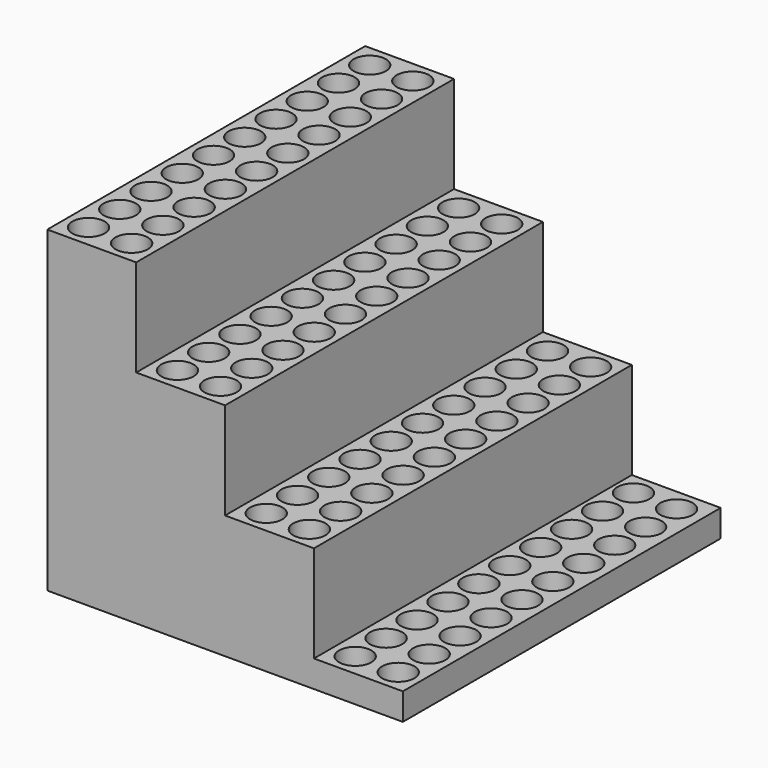
from build123d import *

# Parameters (mm, degrees)
F1_DEPTH  = 295
F2_R      = 12
F3_DEPTH  = 18
F4_R      = 12
F5_DEPTH  = 18
F6_R      = 12
F7_DEPTH  = 18
F8_R      = 12
F9_DEPTH  = 18
F11_DEPTH = 180
F13_DEPTH = 116
F15_DEPTH = 50
F16_DEPTH = 50
F17_DEPTH = 116
F18_DEPTH = 182


# Not quite as in the source:
# - a feature names something its author has since deleted; it is built from what else it names


with BuildPart() as f1:
    # F0 (on Front) → F1 (new body)
    with BuildSketch(Plane.XZ):
        Polygon((-130.714428395, 109.3473359393), (-130.714428395, -126.6526640607), (133.285571605, -126.6526640607), (133.285571605, -106.6526640607), (67.285571605, -106.6526640607), (67.285571605, -34.6526640607), (1.285571605, -34.6526640607), (1.285571605, 37.3473359393), (-64.714428395, 37.3473359393), (-64.714428395, 109.3473359393), align=None)
    extrude(amount=F1_DEPTH)

    # F2 (on face) → F3 (cut)
    with BuildSketch(Plane.XY.offset(-106.6526640607)):
        with Locations((84.285571605, -278)):
            Circle(F2_R)
        with Locations((84.0420044155, -249.0010228624)):
            Circle(F2_R)
        with Locations((83.7984372259, -220.0020457249)):
            Circle(F2_R)
        with Locations((83.5548700364, -191.0030685873)):
            Circle(F2_R)
        with Locations((83.3113028469, -162.0040914498)):
            Circle(F2_R)
        with Locations((83.0677356574, -133.0051143122)):
            Circle(F2_R)
        with Locations((82.8241684679, -104.0061371747)):
            Circle(F2_R)
        with Locations((82.5806012783, -75.0071600371)):
            Circle(F2_R)
        with Locations((82.3370340888, -46.0081828996)):
            Circle(F2_R)
        with Locations((82.0934668993, -17.009205762)):
            Circle(F2_R)
        with Locations((114.0934668993, -17.009205762)):
            Circle(F2_R)
        with Locations((114.3370340888, -46.0081828996)):
            Circle(F2_R)
        with Locations((114.5806012783, -75.0071600371)):
            Circle(F2_R)
        with Locations((114.8241684679, -104.0061371747)):
            Circle(F2_R)
        with Locations((115.0677356574, -133.0051143122)):
            Circle(F2_R)
        with Locations((115.3113028469, -162.0040914498)):
            Circle(F2_R)
        with Locations((115.5548700364, -191.0030685873)):
            Circle(F2_R)
        with Locations((115.7984372259, -220.0020457249)):
            Circle(F2_R)
        with Locations((116.0420044155, -249.0010228624)):
            Circle(F2_R)
        with Locations((116.285571605, -278)):
            Circle(F2_R)
    extrude(amount=-F3_DEPTH, mode=Mode.SUBTRACT)

    # F4 (on face) → F5 (cut)
    with BuildSketch(Plane.XY.offset(-34.6526640607)):
        with Locations((18.285571605, -278)):
            Circle(F4_R)
        with Locations((18.285571605, -249)):
            Circle(F4_R)
        with Locations((18.285571605, -220)):
            Circle(F4_R)
        with Locations((18.285571605, -191)):
            Circle(F4_R)
        with Locations((18.285571605, -162)):
            Circle(F4_R)
        with Locations((18.285571605, -133)):
            Circle(F4_R)
        with Locations((18.285571605, -104)):
            Circle(F4_R)
        with Locations((18.285571605, -75)):
            Circle(F4_R)
        with Locations((18.285571605, -46)):
            Circle(F4_R)
        with Locations((18.285571605, -17)):
            Circle(F4_R)
        with Locations((50.285571605, -17)):
            Circle(F4_R)
        with Locations((50.285571605, -46)):
            Circle(F4_R)
        with Locations((50.285571605, -75)):
            Circle(F4_R)
        with Locations((50.285571605, -104)):
            Circle(F4_R)
        with Locations((50.285571605, -133)):
            Circle(F4_R)
        with Locations((50.285571605, -162)):
            Circle(F4_R)
        with Locations((50.285571605, -191)):
            Circle(F4_R)
        with Locations((50.285571605, -220)):
            Circle(F4_R)
        with Locations((50.285571605, -249)):
            Circle(F4_R)
        with Locations((50.285571605, -278)):
            Circle(F4_R)
    extrude(amount=-F5_DEPTH, mode=Mode.SUBTRACT)

    # F6 (on face) → F7 (cut)
    with BuildSketch(Plane.XY.offset(37.3473359393)):
        with Locations((-47.714428395, -278)):
            Circle(F6_R)
        with Locations((-47.714428395, -249)):
            Circle(F6_R)
        with Locations((-47.714428395, -220)):
            Circle(F6_R)
        with Locations((-47.714428395, -191)):
            Circle(F6_R)
        with Locations((-47.714428395, -162)):
            Circle(F6_R)
        with Locations((-47.714428395, -133)):
            Circle(F6_R)
        with Locations((-47.714428395, -104)):
            Circle(F6_R)
        with Locations((-47.714428395, -75)):
            Circle(F6_R)
        with Locations((-47.714428395, -46)):
            Circle(F6_R)
        with Locations((-47.714428395, -17)):
            Circle(F6_R)
        with Locations((-15.714428395, -17)):
            Circle(F6_R)
        with Locations((-15.714428395, -46)):
            Circle(F6_R)
        with Locations((-15.714428395, -75)):
            Circle(F6_R)
        with Locations((-15.714428395, -104)):
            Circle(F6_R)
        with Locations((-15.714428395, -133)):
            Circle(F6_R)
        with Locations((-15.714428395, -162)):
            Circle(F6_R)
        with Locations((-15.714428395, -191)):
            Circle(F6_R)
        with Locations((-15.714428395, -220)):
            Circle(F6_R)
        with Locations((-15.714428395, -249)):
            Circle(F6_R)
        with Locations((-15.714428395, -278)):
            Circle(F6_R)
    extrude(amount=-F7_DEPTH, mode=Mode.SUBTRACT)

    # F8 (on face) → F9 (cut)
    with BuildSketch(Plane.XY.offset(109.3473359393)):
        with Locations((-113.714428395, -278)):
            Circle(F8_R)
        with Locations((-113.714428395, -249)):
            Circle(F8_R)
        with Locations((-113.714428395, -220)):
            Circle(F8_R)
        with Locations((-113.714428395, -191)):
            Circle(F8_R)
        with Locations((-113.714428395, -162)):
            Circle(F8_R)
        with Locations((-113.714428395, -133)):
            Circle(F8_R)
        with Locations((-113.714428395, -104)):
            Circle(F8_R)
        with Locations((-113.714428395, -75)):
            Circle(F8_R)
        with Locations((-113.714428395, -46)):
            Circle(F8_R)
        with Locations((-113.714428395, -17)):
            Circle(F8_R)
        with Locations((-81.714428395, -17)):
            Circle(F8_R)
        with Locations((-81.714428395, -46)):
            Circle(F8_R)
        with Locations((-81.714428395, -75)):
            Circle(F8_R)
        with Locations((-81.714428395, -104)):
            Circle(F8_R)
        with Locations((-81.714428395, -133)):
            Circle(F8_R)
        with Locations((-81.714428395, -162)):
            Circle(F8_R)
        with Locations((-81.714428395, -191)):
            Circle(F8_R)
        with Locations((-81.714428395, -220)):
            Circle(F8_R)
        with Locations((-81.714428395, -249)):
            Circle(F8_R)
        with Locations((-81.714428395, -278)):
            Circle(F8_R)
    extrude(amount=-F9_DEPTH, mode=Mode.SUBTRACT)

    # F10 (on face) → F11 (cut)
    with BuildSketch(Plane(origin=(-130.714428395, 0, 0), x_dir=(0, -1, 0), z_dir=(-1, 0, 0))):
        with BuildLine():
            ThreePointArc((7.2532056552, -79.6526640607), (17, -84.6526640607), (26.7467943448, -79.6526640607))
            ThreePointArc((26.7467943448, -79.6526640607), (17, -74.6526640607), (7.2532056552, -79.6526640607))
        make_face()
        with BuildLine():
            ThreePointArc((7.2532056552, -79.6526640607), (13.3231489109, -98.0754818422), (29, -86.6526640607))
            ThreePointArc((29, -86.6526640607), (28.4228177815, -82.9758129716), (26.7467943448, -79.6526640607))
            ThreePointArc((26.7467943448, -79.6526640607), (17, -84.6526640607), (7.2532056552, -79.6526640607))
        make_face()
        with BuildLine():
            ThreePointArc((36.2532056552, -79.6526640607), (46, -84.6526640607), (55.7467943448, -79.6526640607))
            ThreePointArc((55.7467943448, -79.6526640607), (46, -74.6526640607), (36.2532056552, -79.6526640607))
        make_face()
        with BuildLine():
            ThreePointArc((36.2532056552, -79.6526640607), (42.3231489109, -98.0754818422), (58, -86.6526640607))
            ThreePointArc((58, -86.6526640607), (57.4228177815, -82.9758129716), (55.7467943448, -79.6526640607))
            ThreePointArc((55.7467943448, -79.6526640607), (46, -84.6526640607), (36.2532056552, -79.6526640607))
        make_face()
        with BuildLine():
            ThreePointArc((65.2532056552, -79.6526640607), (75, -84.6526640607), (84.7467943448, -79.6526640607))
            ThreePointArc((84.7467943448, -79.6526640607), (75, -74.6526640607), (65.2532056552, -79.6526640607))
        make_face()
        with BuildLine():
            ThreePointArc((65.2532056552, -79.6526640607), (71.3231489109, -98.0754818422), (87, -86.6526640607))
            ThreePointArc((87, -86.6526640607), (86.4228177815, -82.9758129716), (84.7467943448, -79.6526640607))
            ThreePointArc((84.7467943448, -79.6526640607), (75, -84.6526640607), (65.2532056552, -79.6526640607))
        make_face()
        with BuildLine():
            ThreePointArc((94.2532056552, -79.6526640607), (104, -84.6526640607), (113.7467943448, -79.6526640607))
            ThreePointArc((113.7467943448, -79.6526640607), (104, -74.6526640607), (94.2532056552, -79.6526640607))
        make_face()
        with BuildLine():
            ThreePointArc((94.2532056552, -79.6526640607), (100.3231489109, -98.0754818422), (116, -86.6526640607))
            ThreePointArc((116, -86.6526640607), (115.4228177815, -82.9758129716), (113.7467943448, -79.6526640607))
            ThreePointArc((113.7467943448, -79.6526640607), (104, -84.6526640607), (94.2532056552, -79.6526640607))
        make_face()
        with BuildLine():
            ThreePointArc((123.2532056552, -79.6526640607), (133, -84.6526640607), (142.7467943448, -79.6526640607))
            ThreePointArc((142.7467943448, -79.6526640607), (133, -74.6526640607), (123.2532056552, -79.6526640607))
        make_face()
        with BuildLine():
            ThreePointArc((123.2532056552, -79.6526640607), (129.3231489109, -98.0754818422), (145, -86.6526640607))
            ThreePointArc((145, -86.6526640607), (144.4228177815, -82.9758129716), (142.7467943448, -79.6526640607))
            ThreePointArc((142.7467943448, -79.6526640607), (133, -84.6526640607), (123.2532056552, -79.6526640607))
        make_face()
        with BuildLine():
            ThreePointArc((152.2532056552, -79.6526640607), (162, -84.6526640607), (171.7467943448, -79.6526640607))
            ThreePointArc((171.7467943448, -79.6526640607), (162, -74.6526640607), (152.2532056552, -79.6526640607))
        make_face()
        with BuildLine():
            ThreePointArc((152.2532056552, -79.6526640607), (158.3231489109, -98.0754818422), (174, -86.6526640607))
            ThreePointArc((174, -86.6526640607), (173.4228177815, -82.9758129716), (171.7467943448, -79.6526640607))
            ThreePointArc((171.7467943448, -79.6526640607), (162, -84.6526640607), (152.2532056552, -79.6526640607))
        make_face()
        with BuildLine():
            ThreePointArc((181.2532056552, -79.6526640607), (191, -84.6526640607), (200.7467943448, -79.6526640607))
            ThreePointArc((200.7467943448, -79.6526640607), (191, -74.6526640607), (181.2532056552, -79.6526640607))
        make_face()
        with BuildLine():
            ThreePointArc((181.2532056552, -79.6526640607), (187.3231489109, -98.0754818422), (203, -86.6526640607))
            ThreePointArc((203, -86.6526640607), (202.4228177815, -82.9758129716), (200.7467943448, -79.6526640607))
            ThreePointArc((200.7467943448, -79.6526640607), (191, -84.6526640607), (181.2532056552, -79.6526640607))
        make_face()
        with BuildLine():
            ThreePointArc((210.2532056552, -79.6526640607), (220, -84.6526640607), (229.7467943448, -79.6526640607))
            ThreePointArc((229.7467943448, -79.6526640607), (220, -74.6526640607), (210.2532056552, -79.6526640607))
        make_face()
        with BuildLine():
            ThreePointArc((210.2532056552, -79.6526640607), (216.3231489109, -98.0754818422), (232, -86.6526640607))
            ThreePointArc((232, -86.6526640607), (231.4228177815, -82.9758129716), (229.7467943448, -79.6526640607))
            ThreePointArc((229.7467943448, -79.6526640607), (220, -84.6526640607), (210.2532056552, -79.6526640607))
        make_face()
        with BuildLine():
            ThreePointArc((239.2532056552, -79.6526640607), (249, -84.6526640607), (258.7467943448, -79.6526640607))
            ThreePointArc((258.7467943448, -79.6526640607), (249, -74.6526640607), (239.2532056552, -79.6526640607))
        make_face()
        with BuildLine():
            ThreePointArc((239.2532056552, -79.6526640607), (245.3231489109, -98.0754818422), (261, -86.6526640607))
            ThreePointArc((261, -86.6526640607), (260.4228177815, -82.9758129716), (258.7467943448, -79.6526640607))
            ThreePointArc((258.7467943448, -79.6526640607), (249, -84.6526640607), (239.2532056552, -79.6526640607))
        make_face()
        with BuildLine():
            ThreePointArc((268.2532056552, -79.6526640607), (278, -84.6526640607), (287.7467943448, -79.6526640607))
            ThreePointArc((287.7467943448, -79.6526640607), (278, -74.6526640607), (268.2532056552, -79.6526640607))
        make_face()
        with BuildLine():
            ThreePointArc((268.2532056552, -79.6526640607), (274.3231489109, -98.0754818422), (290, -86.6526640607))
            ThreePointArc((290, -86.6526640607), (289.4228177815, -82.9758129716), (287.7467943448, -79.6526640607))
            ThreePointArc((287.7467943448, -79.6526640607), (278, -84.6526640607), (268.2532056552, -79.6526640607))
        make_face()
    extrude(amount=-F11_DEPTH, mode=Mode.SUBTRACT)

    # F12 (on face) → F13 (cut)
    with BuildSketch(Plane(origin=(-130.714428395, 0, 0), x_dir=(0, -1, 0), z_dir=(-1, 0, 0))):
        with BuildLine():
            ThreePointArc((7.2532056552, -3.6526640607), (17, -8.6526640607), (26.7467943448, -3.6526640607))
            ThreePointArc((26.7467943448, -3.6526640607), (17, 1.3473359393), (7.2532056552, -3.6526640607))
        make_face()
        with BuildLine():
            ThreePointArc((7.2532056552, -3.6526640607), (13.3231489109, -22.0754818422), (29, -10.6526640607))
            ThreePointArc((29, -10.6526640607), (28.4228177815, -6.9758129716), (26.7467943448, -3.6526640607))
            ThreePointArc((26.7467943448, -3.6526640607), (17, -8.6526640607), (7.2532056552, -3.6526640607))
        make_face()
        with BuildLine():
            ThreePointArc((36.2532056552, -3.6526640607), (46, -8.6526640607), (55.7467943448, -3.6526640607))
            ThreePointArc((55.7467943448, -3.6526640607), (46, 1.3473359393), (36.2532056552, -3.6526640607))
        make_face()
        with BuildLine():
            ThreePointArc((36.2532056552, -3.6526640607), (42.3231489109, -22.0754818422), (58, -10.6526640607))
            ThreePointArc((58, -10.6526640607), (57.4228177815, -6.9758129716), (55.7467943448, -3.6526640607))
            ThreePointArc((55.7467943448, -3.6526640607), (46, -8.6526640607), (36.2532056552, -3.6526640607))
        make_face()
        with BuildLine():
            ThreePointArc((65.2532056552, -3.6526640607), (75, -8.6526640607), (84.7467943448, -3.6526640607))
            ThreePointArc((84.7467943448, -3.6526640607), (75, 1.3473359393), (65.2532056552, -3.6526640607))
        make_face()
        with BuildLine():
            ThreePointArc((65.2532056552, -3.6526640607), (71.3231489109, -22.0754818422), (87, -10.6526640607))
            ThreePointArc((87, -10.6526640607), (86.4228177815, -6.9758129716), (84.7467943448, -3.6526640607))
            ThreePointArc((84.7467943448, -3.6526640607), (75, -8.6526640607), (65.2532056552, -3.6526640607))
        make_face()
        with BuildLine():
            ThreePointArc((94.2532056552, -3.6526640607), (104, -8.6526640607), (113.7467943448, -3.6526640607))
            ThreePointArc((113.7467943448, -3.6526640607), (104, 1.3473359393), (94.2532056552, -3.6526640607))
        make_face()
        with BuildLine():
            ThreePointArc((94.2532056552, -3.6526640607), (100.3231489109, -22.0754818422), (116, -10.6526640607))
            ThreePointArc((116, -10.6526640607), (115.4228177815, -6.9758129716), (113.7467943448, -3.6526640607))
            ThreePointArc((113.7467943448, -3.6526640607), (104, -8.6526640607), (94.2532056552, -3.6526640607))
        make_face()
        with BuildLine():
            ThreePointArc((123.2532056552, -3.6526640607), (133, -8.6526640607), (142.7467943448, -3.6526640607))
            ThreePointArc((142.7467943448, -3.6526640607), (133, 1.3473359393), (123.2532056552, -3.6526640607))
        make_face()
        with BuildLine():
            ThreePointArc((123.2532056552, -3.6526640607), (129.3231489109, -22.0754818422), (145, -10.6526640607))
            ThreePointArc((145, -10.6526640607), (144.4228177815, -6.9758129716), (142.7467943448, -3.6526640607))
            ThreePointArc((142.7467943448, -3.6526640607), (133, -8.6526640607), (123.2532056552, -3.6526640607))
        make_face()
        with BuildLine():
            ThreePointArc((152.2532056552, -3.6526640607), (162, -8.6526640607), (171.7467943448, -3.6526640607))
            ThreePointArc((171.7467943448, -3.6526640607), (162, 1.3473359393), (152.2532056552, -3.6526640607))
        make_face()
        with BuildLine():
            ThreePointArc((152.2532056552, -3.6526640607), (158.3231489109, -22.0754818422), (174, -10.6526640607))
            ThreePointArc((174, -10.6526640607), (173.4228177815, -6.9758129716), (171.7467943448, -3.6526640607))
            ThreePointArc((171.7467943448, -3.6526640607), (162, -8.6526640607), (152.2532056552, -3.6526640607))
        make_face()
        with BuildLine():
            ThreePointArc((181.2532056552, -3.6526640607), (191, -8.6526640607), (200.7467943448, -3.6526640607))
            ThreePointArc((200.7467943448, -3.6526640607), (191, 1.3473359393), (181.2532056552, -3.6526640607))
        make_face()
        with BuildLine():
            ThreePointArc((181.2532056552, -3.6526640607), (187.3231489109, -22.0754818422), (203, -10.6526640607))
            ThreePointArc((203, -10.6526640607), (202.4228177815, -6.9758129716), (200.7467943448, -3.6526640607))
            ThreePointArc((200.7467943448, -3.6526640607), (191, -8.6526640607), (181.2532056552, -3.6526640607))
        make_face()
        with BuildLine():
            ThreePointArc((210.2532056552, -3.6526640607), (220, -8.6526640607), (229.7467943448, -3.6526640607))
            ThreePointArc((229.7467943448, -3.6526640607), (220, 1.3473359393), (210.2532056552, -3.6526640607))
        make_face()
        with BuildLine():
            ThreePointArc((210.2532056552, -3.6526640607), (216.3231489109, -22.0754818422), (232, -10.6526640607))
            ThreePointArc((232, -10.6526640607), (231.4228177815, -6.9758129716), (229.7467943448, -3.6526640607))
            ThreePointArc((229.7467943448, -3.6526640607), (220, -8.6526640607), (210.2532056552, -3.6526640607))
        make_face()
        with BuildLine():
            ThreePointArc((239.2532056552, -3.6526640607), (249, -8.6526640607), (258.7467943448, -3.6526640607))
            ThreePointArc((258.7467943448, -3.6526640607), (249, 1.3473359393), (239.2532056552, -3.6526640607))
        make_face()
        with BuildLine():
            ThreePointArc((239.2532056552, -3.6526640607), (245.3231489109, -22.0754818422), (261, -10.6526640607))
            ThreePointArc((261, -10.6526640607), (260.4228177815, -6.9758129716), (258.7467943448, -3.6526640607))
            ThreePointArc((258.7467943448, -3.6526640607), (249, -8.6526640607), (239.2532056552, -3.6526640607))
        make_face()
        with BuildLine():
            ThreePointArc((268.2532056552, -3.6526640607), (278, -8.6526640607), (287.7467943448, -3.6526640607))
            ThreePointArc((287.7467943448, -3.6526640607), (278, 1.3473359393), (268.2532056552, -3.6526640607))
        make_face()
        with BuildLine():
            ThreePointArc((268.2532056552, -3.6526640607), (274.3231489109, -22.0754818422), (290, -10.6526640607))
            ThreePointArc((290, -10.6526640607), (289.4228177815, -6.9758129716), (287.7467943448, -3.6526640607))
            ThreePointArc((287.7467943448, -3.6526640607), (278, -8.6526640607), (268.2532056552, -3.6526640607))
        make_face()
    extrude(amount=-F13_DEPTH, mode=Mode.SUBTRACT)

    # F14 (on face) → F15 (cut)
    with BuildSketch(Plane(origin=(-130.714428395, 0, 0), x_dir=(0, -1, 0), z_dir=(-1, 0, 0))):
        with BuildLine():
            ThreePointArc((7.6342224749, 65.8215485745), (16.3479186261, 61.3414258771), (25.4963356933, 64.8494830553))
            ThreePointArc((25.4963356933, 64.8494830553), (16.782639542, 69.3296057527), (7.6342224749, 65.8215485745))
        make_face()
        with BuildLine():
            ThreePointArc((7.6342224749, 65.8215485745), (11.5455842489, 46.2577906754), (28.1305581682, 57.3473359393))
            ThreePointArc((28.1305581682, 57.3473359393), (27.4528664642, 61.322928329), (25.4963356933, 64.8494830553))
            ThreePointArc((25.4963356933, 64.8494830553), (16.3479186261, 61.3414258771), (7.6342224749, 65.8215485745))
        make_face()
        with BuildLine():
            ThreePointArc((36.6342224749, 65.8215485745), (45.3479186261, 61.3414258771), (54.4963356933, 64.8494830553))
            ThreePointArc((54.4963356933, 64.8494830553), (45.782639542, 69.3296057527), (36.6342224749, 65.8215485745))
        make_face()
        with BuildLine():
            ThreePointArc((36.6342224749, 65.8215485745), (40.5455842489, 46.2577906754), (57.1305581682, 57.3473359393))
            ThreePointArc((57.1305581682, 57.3473359393), (56.4528664642, 61.322928329), (54.4963356933, 64.8494830553))
            ThreePointArc((54.4963356933, 64.8494830553), (45.3479186261, 61.3414258771), (36.6342224749, 65.8215485745))
        make_face()
        with BuildLine():
            ThreePointArc((65.6342224749, 65.8215485745), (74.3479186261, 61.3414258771), (83.4963356933, 64.8494830553))
            ThreePointArc((83.4963356933, 64.8494830553), (74.782639542, 69.3296057527), (65.6342224749, 65.8215485745))
        make_face()
        with BuildLine():
            ThreePointArc((65.6342224749, 65.8215485745), (69.5455842489, 46.2577906754), (86.1305581682, 57.3473359393))
            ThreePointArc((86.1305581682, 57.3473359393), (85.4528664642, 61.322928329), (83.4963356933, 64.8494830553))
            ThreePointArc((83.4963356933, 64.8494830553), (74.3479186261, 61.3414258771), (65.6342224749, 65.8215485745))
        make_face()
        with BuildLine():
            ThreePointArc((94.6342224749, 65.8215485745), (103.3479186261, 61.3414258771), (112.4963356933, 64.8494830553))
            ThreePointArc((112.4963356933, 64.8494830553), (103.782639542, 69.3296057527), (94.6342224749, 65.8215485745))
        make_face()
        with BuildLine():
            ThreePointArc((94.6342224749, 65.8215485745), (98.5455842489, 46.2577906754), (115.1305581682, 57.3473359393))
            ThreePointArc((115.1305581682, 57.3473359393), (114.4528664642, 61.322928329), (112.4963356933, 64.8494830553))
            ThreePointArc((112.4963356933, 64.8494830553), (103.3479186261, 61.3414258771), (94.6342224749, 65.8215485745))
        make_face()
        with BuildLine():
            ThreePointArc((123.6342224749, 65.8215485745), (132.3479186261, 61.3414258771), (141.4963356933, 64.8494830553))
            ThreePointArc((141.4963356933, 64.8494830553), (132.782639542, 69.3296057527), (123.6342224749, 65.8215485745))
        make_face()
        with BuildLine():
            ThreePointArc((123.6342224749, 65.8215485745), (127.5455842489, 46.2577906754), (144.1305581682, 57.3473359393))
            ThreePointArc((144.1305581682, 57.3473359393), (143.4528664642, 61.322928329), (141.4963356933, 64.8494830553))
            ThreePointArc((141.4963356933, 64.8494830553), (132.3479186261, 61.3414258771), (123.6342224749, 65.8215485745))
        make_face()
        with BuildLine():
            ThreePointArc((152.6342224749, 65.8215485745), (161.3479186261, 61.3414258771), (170.4963356933, 64.8494830553))
            ThreePointArc((170.4963356933, 64.8494830553), (161.782639542, 69.3296057527), (152.6342224749, 65.8215485745))
        make_face()
        with BuildLine():
            ThreePointArc((152.6342224749, 65.8215485745), (156.5455842489, 46.2577906754), (173.1305581682, 57.3473359393))
            ThreePointArc((173.1305581682, 57.3473359393), (172.4528664642, 61.322928329), (170.4963356933, 64.8494830553))
            ThreePointArc((170.4963356933, 64.8494830553), (161.3479186261, 61.3414258771), (152.6342224749, 65.8215485745))
        make_face()
        with BuildLine():
            ThreePointArc((181.6342224749, 65.8215485745), (190.3479186261, 61.3414258771), (199.4963356933, 64.8494830553))
            ThreePointArc((199.4963356933, 64.8494830553), (190.782639542, 69.3296057527), (181.6342224749, 65.8215485745))
        make_face()
        with BuildLine():
            ThreePointArc((181.6342224749, 65.8215485745), (185.5455842489, 46.2577906754), (202.1305581682, 57.3473359393))
            ThreePointArc((202.1305581682, 57.3473359393), (201.4528664642, 61.322928329), (199.4963356933, 64.8494830553))
            ThreePointArc((199.4963356933, 64.8494830553), (190.3479186261, 61.3414258771), (181.6342224749, 65.8215485745))
        make_face()
        with BuildLine():
            ThreePointArc((210.6342224749, 65.8215485745), (219.3479186261, 61.3414258771), (228.4963356933, 64.8494830553))
            ThreePointArc((228.4963356933, 64.8494830553), (219.782639542, 69.3296057527), (210.6342224749, 65.8215485745))
        make_face()
        with BuildLine():
            ThreePointArc((210.6342224749, 65.8215485745), (214.5455842489, 46.2577906754), (231.1305581682, 57.3473359393))
            ThreePointArc((231.1305581682, 57.3473359393), (230.4528664642, 61.322928329), (228.4963356933, 64.8494830553))
            ThreePointArc((228.4963356933, 64.8494830553), (219.3479186261, 61.3414258771), (210.6342224749, 65.8215485745))
        make_face()
        with BuildLine():
            ThreePointArc((239.6342224749, 65.8215485745), (248.3479186261, 61.3414258771), (257.4963356933, 64.8494830553))
            ThreePointArc((257.4963356933, 64.8494830553), (248.782639542, 69.3296057527), (239.6342224749, 65.8215485745))
        make_face()
        with BuildLine():
            ThreePointArc((239.6342224749, 65.8215485745), (243.5455842489, 46.2577906754), (260.1305581682, 57.3473359393))
            ThreePointArc((260.1305581682, 57.3473359393), (259.4528664642, 61.322928329), (257.4963356933, 64.8494830553))
            ThreePointArc((257.4963356933, 64.8494830553), (248.3479186261, 61.3414258771), (239.6342224749, 65.8215485745))
        make_face()
        with BuildLine():
            ThreePointArc((268.6342224749, 65.8215485745), (277.3479186261, 61.3414258771), (286.4963356933, 64.8494830553))
            ThreePointArc((286.4963356933, 64.8494830553), (277.782639542, 69.3296057527), (268.6342224749, 65.8215485745))
        make_face()
        with BuildLine():
            ThreePointArc((268.6342224749, 65.8215485745), (272.5455842489, 46.2577906754), (289.1305581682, 57.3473359393))
            ThreePointArc((289.1305581682, 57.3473359393), (288.4528664642, 61.322928329), (286.4963356933, 64.8494830553))
            ThreePointArc((286.4963356933, 64.8494830553), (277.3479186261, 61.3414258771), (268.6342224749, 65.8215485745))
        make_face()
    extrude(amount=-F15_DEPTH, mode=Mode.SUBTRACT)

    # F14 (on face) → F16 (cut)
    with BuildSketch(Plane(origin=(-130.714428395, 0, 0), x_dir=(0, -1, 0), z_dir=(-1, 0, 0))):
        with BuildLine():
            ThreePointArc((7.6342224749, 65.8215485745), (11.5455842489, 46.2577906754), (28.1305581682, 57.3473359393))
            ThreePointArc((28.1305581682, 57.3473359393), (27.4528664642, 61.322928329), (25.4963356933, 64.8494830553))
            ThreePointArc((25.4963356933, 64.8494830553), (16.3479186261, 61.3414258771), (7.6342224749, 65.8215485745))
        make_face()
        with BuildLine():
            ThreePointArc((7.6342224749, 65.8215485745), (16.3479186261, 61.3414258771), (25.4963356933, 64.8494830553))
            ThreePointArc((25.4963356933, 64.8494830553), (16.782639542, 69.3296057527), (7.6342224749, 65.8215485745))
        make_face()
        with BuildLine():
            ThreePointArc((7.6342224749, 65.8215485745), (16.782639542, 69.3296057527), (25.4963356933, 64.8494830553))
            ThreePointArc((25.4963356933, 64.8494830553), (28.0895452639, 68.7387217713), (29, 73.3236956905))
            ThreePointArc((29, 73.3236956905), (13.0244076103, 84.6460039866), (7.6342224749, 65.8215485745))
        make_face()
        with BuildLine():
            ThreePointArc((36.6342224749, 65.8215485745), (40.5455842489, 46.2577906754), (57.1305581682, 57.3473359393))
            ThreePointArc((57.1305581682, 57.3473359393), (56.4528664642, 61.322928329), (54.4963356933, 64.8494830553))
            ThreePointArc((54.4963356933, 64.8494830553), (45.3479186261, 61.3414258771), (36.6342224749, 65.8215485745))
        make_face()
        with BuildLine():
            ThreePointArc((36.6342224749, 65.8215485745), (45.3479186261, 61.3414258771), (54.4963356933, 64.8494830553))
            ThreePointArc((54.4963356933, 64.8494830553), (45.782639542, 69.3296057527), (36.6342224749, 65.8215485745))
        make_face()
        with BuildLine():
            ThreePointArc((36.6342224749, 65.8215485745), (45.782639542, 69.3296057527), (54.4963356933, 64.8494830553))
            ThreePointArc((54.4963356933, 64.8494830553), (57.0895452639, 68.7387217713), (58, 73.3236956905))
            ThreePointArc((58, 73.3236956905), (42.0244076103, 84.6460039866), (36.6342224749, 65.8215485745))
        make_face()
        with BuildLine():
            ThreePointArc((65.6342224749, 65.8215485745), (69.5455842489, 46.2577906754), (86.1305581682, 57.3473359393))
            ThreePointArc((86.1305581682, 57.3473359393), (85.4528664642, 61.322928329), (83.4963356933, 64.8494830553))
            ThreePointArc((83.4963356933, 64.8494830553), (74.3479186261, 61.3414258771), (65.6342224749, 65.8215485745))
        make_face()
        with BuildLine():
            ThreePointArc((65.6342224749, 65.8215485745), (74.3479186261, 61.3414258771), (83.4963356933, 64.8494830553))
            ThreePointArc((83.4963356933, 64.8494830553), (74.782639542, 69.3296057527), (65.6342224749, 65.8215485745))
        make_face()
        with BuildLine():
            ThreePointArc((65.6342224749, 65.8215485745), (74.782639542, 69.3296057527), (83.4963356933, 64.8494830553))
            ThreePointArc((83.4963356933, 64.8494830553), (86.0895452639, 68.7387217713), (87, 73.3236956905))
            ThreePointArc((87, 73.3236956905), (71.0244076103, 84.6460039866), (65.6342224749, 65.8215485745))
        make_face()
        with BuildLine():
            ThreePointArc((94.6342224749, 65.8215485745), (98.5455842489, 46.2577906754), (115.1305581682, 57.3473359393))
            ThreePointArc((115.1305581682, 57.3473359393), (114.4528664642, 61.322928329), (112.4963356933, 64.8494830553))
            ThreePointArc((112.4963356933, 64.8494830553), (103.3479186261, 61.3414258771), (94.6342224749, 65.8215485745))
        make_face()
        with BuildLine():
            ThreePointArc((94.6342224749, 65.8215485745), (103.3479186261, 61.3414258771), (112.4963356933, 64.8494830553))
            ThreePointArc((112.4963356933, 64.8494830553), (103.782639542, 69.3296057527), (94.6342224749, 65.8215485745))
        make_face()
        with BuildLine():
            ThreePointArc((94.6342224749, 65.8215485745), (103.782639542, 69.3296057527), (112.4963356933, 64.8494830553))
            ThreePointArc((112.4963356933, 64.8494830553), (115.0895452639, 68.7387217713), (116, 73.3236956905))
            ThreePointArc((116, 73.3236956905), (100.0244076103, 84.6460039866), (94.6342224749, 65.8215485745))
        make_face()
        with BuildLine():
            ThreePointArc((123.6342224749, 65.8215485745), (127.5455842489, 46.2577906754), (144.1305581682, 57.3473359393))
            ThreePointArc((144.1305581682, 57.3473359393), (143.4528664642, 61.322928329), (141.4963356933, 64.8494830553))
            ThreePointArc((141.4963356933, 64.8494830553), (132.3479186261, 61.3414258771), (123.6342224749, 65.8215485745))
        make_face()
        with BuildLine():
            ThreePointArc((123.6342224749, 65.8215485745), (132.3479186261, 61.3414258771), (141.4963356933, 64.8494830553))
            ThreePointArc((141.4963356933, 64.8494830553), (132.782639542, 69.3296057527), (123.6342224749, 65.8215485745))
        make_face()
        with BuildLine():
            ThreePointArc((123.6342224749, 65.8215485745), (132.782639542, 69.3296057527), (141.4963356933, 64.8494830553))
            ThreePointArc((141.4963356933, 64.8494830553), (144.0895452639, 68.7387217713), (145, 73.3236956905))
            ThreePointArc((145, 73.3236956905), (129.0244076103, 84.6460039866), (123.6342224749, 65.8215485745))
        make_face()
        with BuildLine():
            ThreePointArc((152.6342224749, 65.8215485745), (156.5455842489, 46.2577906754), (173.1305581682, 57.3473359393))
            ThreePointArc((173.1305581682, 57.3473359393), (172.4528664642, 61.322928329), (170.4963356933, 64.8494830553))
            ThreePointArc((170.4963356933, 64.8494830553), (161.3479186261, 61.3414258771), (152.6342224749, 65.8215485745))
        make_face()
        with BuildLine():
            ThreePointArc((152.6342224749, 65.8215485745), (161.3479186261, 61.3414258771), (170.4963356933, 64.8494830553))
            ThreePointArc((170.4963356933, 64.8494830553), (161.782639542, 69.3296057527), (152.6342224749, 65.8215485745))
        make_face()
        with BuildLine():
            ThreePointArc((152.6342224749, 65.8215485745), (161.782639542, 69.3296057527), (170.4963356933, 64.8494830553))
            ThreePointArc((170.4963356933, 64.8494830553), (173.0895452639, 68.7387217713), (174, 73.3236956905))
            ThreePointArc((174, 73.3236956905), (158.0244076103, 84.6460039866), (152.6342224749, 65.8215485745))
        make_face()
        with BuildLine():
            ThreePointArc((181.6342224749, 65.8215485745), (185.5455842489, 46.2577906754), (202.1305581682, 57.3473359393))
            ThreePointArc((202.1305581682, 57.3473359393), (201.4528664642, 61.322928329), (199.4963356933, 64.8494830553))
            ThreePointArc((199.4963356933, 64.8494830553), (190.3479186261, 61.3414258771), (181.6342224749, 65.8215485745))
        make_face()
        with BuildLine():
            ThreePointArc((181.6342224749, 65.8215485745), (190.3479186261, 61.3414258771), (199.4963356933, 64.8494830553))
            ThreePointArc((199.4963356933, 64.8494830553), (190.782639542, 69.3296057527), (181.6342224749, 65.8215485745))
        make_face()
        with BuildLine():
            ThreePointArc((181.6342224749, 65.8215485745), (190.782639542, 69.3296057527), (199.4963356933, 64.8494830553))
            ThreePointArc((199.4963356933, 64.8494830553), (202.0895452639, 68.7387217713), (203, 73.3236956905))
            ThreePointArc((203, 73.3236956905), (187.0244076103, 84.6460039866), (181.6342224749, 65.8215485745))
        make_face()
        with BuildLine():
            ThreePointArc((210.6342224749, 65.8215485745), (214.5455842489, 46.2577906754), (231.1305581682, 57.3473359393))
            ThreePointArc((231.1305581682, 57.3473359393), (230.4528664642, 61.322928329), (228.4963356933, 64.8494830553))
            ThreePointArc((228.4963356933, 64.8494830553), (219.3479186261, 61.3414258771), (210.6342224749, 65.8215485745))
        make_face()
        with BuildLine():
            ThreePointArc((210.6342224749, 65.8215485745), (219.3479186261, 61.3414258771), (228.4963356933, 64.8494830553))
            ThreePointArc((228.4963356933, 64.8494830553), (219.782639542, 69.3296057527), (210.6342224749, 65.8215485745))
        make_face()
        with BuildLine():
            ThreePointArc((210.6342224749, 65.8215485745), (219.782639542, 69.3296057527), (228.4963356933, 64.8494830553))
            ThreePointArc((228.4963356933, 64.8494830553), (231.0895452639, 68.7387217713), (232, 73.3236956905))
            ThreePointArc((232, 73.3236956905), (216.0244076103, 84.6460039866), (210.6342224749, 65.8215485745))
        make_face()
        with BuildLine():
            ThreePointArc((239.6342224749, 65.8215485745), (243.5455842489, 46.2577906754), (260.1305581682, 57.3473359393))
            ThreePointArc((260.1305581682, 57.3473359393), (259.4528664642, 61.322928329), (257.4963356933, 64.8494830553))
            ThreePointArc((257.4963356933, 64.8494830553), (248.3479186261, 61.3414258771), (239.6342224749, 65.8215485745))
        make_face()
        with BuildLine():
            ThreePointArc((239.6342224749, 65.8215485745), (248.3479186261, 61.3414258771), (257.4963356933, 64.8494830553))
            ThreePointArc((257.4963356933, 64.8494830553), (248.782639542, 69.3296057527), (239.6342224749, 65.8215485745))
        make_face()
        with BuildLine():
            ThreePointArc((239.6342224749, 65.8215485745), (248.782639542, 69.3296057527), (257.4963356933, 64.8494830553))
            ThreePointArc((257.4963356933, 64.8494830553), (260.0895452639, 68.7387217713), (261, 73.3236956905))
            ThreePointArc((261, 73.3236956905), (245.0244076103, 84.6460039866), (239.6342224749, 65.8215485745))
        make_face()
        with BuildLine():
            ThreePointArc((268.6342224749, 65.8215485745), (272.5455842489, 46.2577906754), (289.1305581682, 57.3473359393))
            ThreePointArc((289.1305581682, 57.3473359393), (288.4528664642, 61.322928329), (286.4963356933, 64.8494830553))
            ThreePointArc((286.4963356933, 64.8494830553), (277.3479186261, 61.3414258771), (268.6342224749, 65.8215485745))
        make_face()
        with BuildLine():
            ThreePointArc((268.6342224749, 65.8215485745), (277.3479186261, 61.3414258771), (286.4963356933, 64.8494830553))
            ThreePointArc((286.4963356933, 64.8494830553), (277.782639542, 69.3296057527), (268.6342224749, 65.8215485745))
        make_face()
        with BuildLine():
            ThreePointArc((268.6342224749, 65.8215485745), (277.782639542, 69.3296057527), (286.4963356933, 64.8494830553))
            ThreePointArc((286.4963356933, 64.8494830553), (289.0895452639, 68.7387217713), (290, 73.3236956905))
            ThreePointArc((290, 73.3236956905), (274.0244076103, 84.6460039866), (268.6342224749, 65.8215485745))
        make_face()
    extrude(amount=-F16_DEPTH, mode=Mode.SUBTRACT)

    # F12 (on face) → F17 (cut)
    with BuildSketch(Plane(origin=(-130.714428395, 0, 0), x_dir=(0, -1, 0), z_dir=(-1, 0, 0))):
        with BuildLine():
            ThreePointArc((7.2532056552, -3.6526640607), (13.3231489109, -22.0754818422), (29, -10.6526640607))
            ThreePointArc((29, -10.6526640607), (28.4228177815, -6.9758129716), (26.7467943448, -3.6526640607))
            ThreePointArc((26.7467943448, -3.6526640607), (17, -8.6526640607), (7.2532056552, -3.6526640607))
        make_face()
        with BuildLine():
            ThreePointArc((7.2532056552, -3.6526640607), (17, -8.6526640607), (26.7467943448, -3.6526640607))
            ThreePointArc((26.7467943448, -3.6526640607), (17, 1.3473359393), (7.2532056552, -3.6526640607))
        make_face()
        with BuildLine():
            ThreePointArc((7.2532056552, -3.6526640607), (17, 1.3473359393), (26.7467943448, -3.6526640607))
            ThreePointArc((26.7467943448, -3.6526640607), (28.4228177815, -0.3295151498), (29, 3.3473359393))
            ThreePointArc((29, 3.3473359393), (13.3231489109, 14.7701537208), (7.2532056552, -3.6526640607))
        make_face()
        with BuildLine():
            ThreePointArc((36.2532056552, -3.6526640607), (42.3231489109, -22.0754818422), (58, -10.6526640607))
            ThreePointArc((58, -10.6526640607), (57.4228177815, -6.9758129716), (55.7467943448, -3.6526640607))
            ThreePointArc((55.7467943448, -3.6526640607), (46, -8.6526640607), (36.2532056552, -3.6526640607))
        make_face()
        with BuildLine():
            ThreePointArc((36.2532056552, -3.6526640607), (46, -8.6526640607), (55.7467943448, -3.6526640607))
            ThreePointArc((55.7467943448, -3.6526640607), (46, 1.3473359393), (36.2532056552, -3.6526640607))
        make_face()
        with BuildLine():
            ThreePointArc((36.2532056552, -3.6526640607), (46, 1.3473359393), (55.7467943448, -3.6526640607))
            ThreePointArc((55.7467943448, -3.6526640607), (57.4228177815, -0.3295151498), (58, 3.3473359393))
            ThreePointArc((58, 3.3473359393), (42.3231489109, 14.7701537208), (36.2532056552, -3.6526640607))
        make_face()
        with BuildLine():
            ThreePointArc((65.2532056552, -3.6526640607), (71.3231489109, -22.0754818422), (87, -10.6526640607))
            ThreePointArc((87, -10.6526640607), (86.4228177815, -6.9758129716), (84.7467943448, -3.6526640607))
            ThreePointArc((84.7467943448, -3.6526640607), (75, -8.6526640607), (65.2532056552, -3.6526640607))
        make_face()
        with BuildLine():
            ThreePointArc((65.2532056552, -3.6526640607), (75, -8.6526640607), (84.7467943448, -3.6526640607))
            ThreePointArc((84.7467943448, -3.6526640607), (75, 1.3473359393), (65.2532056552, -3.6526640607))
        make_face()
        with BuildLine():
            ThreePointArc((65.2532056552, -3.6526640607), (75, 1.3473359393), (84.7467943448, -3.6526640607))
            ThreePointArc((84.7467943448, -3.6526640607), (86.4228177815, -0.3295151498), (87, 3.3473359393))
            ThreePointArc((87, 3.3473359393), (71.3231489109, 14.7701537208), (65.2532056552, -3.6526640607))
        make_face()
        with BuildLine():
            ThreePointArc((94.2532056552, -3.6526640607), (100.3231489109, -22.0754818422), (116, -10.6526640607))
            ThreePointArc((116, -10.6526640607), (115.4228177815, -6.9758129716), (113.7467943448, -3.6526640607))
            ThreePointArc((113.7467943448, -3.6526640607), (104, -8.6526640607), (94.2532056552, -3.6526640607))
        make_face()
        with BuildLine():
            ThreePointArc((94.2532056552, -3.6526640607), (104, -8.6526640607), (113.7467943448, -3.6526640607))
            ThreePointArc((113.7467943448, -3.6526640607), (104, 1.3473359393), (94.2532056552, -3.6526640607))
        make_face()
        with BuildLine():
            ThreePointArc((94.2532056552, -3.6526640607), (104, 1.3473359393), (113.7467943448, -3.6526640607))
            ThreePointArc((113.7467943448, -3.6526640607), (115.4228177815, -0.3295151498), (116, 3.3473359393))
            ThreePointArc((116, 3.3473359393), (100.3231489109, 14.7701537208), (94.2532056552, -3.6526640607))
        make_face()
        with BuildLine():
            ThreePointArc((123.2532056552, -3.6526640607), (129.3231489109, -22.0754818422), (145, -10.6526640607))
            ThreePointArc((145, -10.6526640607), (144.4228177815, -6.9758129716), (142.7467943448, -3.6526640607))
            ThreePointArc((142.7467943448, -3.6526640607), (133, -8.6526640607), (123.2532056552, -3.6526640607))
        make_face()
        with BuildLine():
            ThreePointArc((123.2532056552, -3.6526640607), (133, -8.6526640607), (142.7467943448, -3.6526640607))
            ThreePointArc((142.7467943448, -3.6526640607), (133, 1.3473359393), (123.2532056552, -3.6526640607))
        make_face()
        with BuildLine():
            ThreePointArc((123.2532056552, -3.6526640607), (133, 1.3473359393), (142.7467943448, -3.6526640607))
            ThreePointArc((142.7467943448, -3.6526640607), (144.4228177815, -0.3295151498), (145, 3.3473359393))
            ThreePointArc((145, 3.3473359393), (129.3231489109, 14.7701537208), (123.2532056552, -3.6526640607))
        make_face()
        with BuildLine():
            ThreePointArc((152.2532056552, -3.6526640607), (158.3231489109, -22.0754818422), (174, -10.6526640607))
            ThreePointArc((174, -10.6526640607), (173.4228177815, -6.9758129716), (171.7467943448, -3.6526640607))
            ThreePointArc((171.7467943448, -3.6526640607), (162, -8.6526640607), (152.2532056552, -3.6526640607))
        make_face()
        with BuildLine():
            ThreePointArc((152.2532056552, -3.6526640607), (162, -8.6526640607), (171.7467943448, -3.6526640607))
            ThreePointArc((171.7467943448, -3.6526640607), (162, 1.3473359393), (152.2532056552, -3.6526640607))
        make_face()
        with BuildLine():
            ThreePointArc((152.2532056552, -3.6526640607), (162, 1.3473359393), (171.7467943448, -3.6526640607))
            ThreePointArc((171.7467943448, -3.6526640607), (173.4228177815, -0.3295151498), (174, 3.3473359393))
            ThreePointArc((174, 3.3473359393), (158.3231489109, 14.7701537208), (152.2532056552, -3.6526640607))
        make_face()
        with BuildLine():
            ThreePointArc((181.2532056552, -3.6526640607), (187.3231489109, -22.0754818422), (203, -10.6526640607))
            ThreePointArc((203, -10.6526640607), (202.4228177815, -6.9758129716), (200.7467943448, -3.6526640607))
            ThreePointArc((200.7467943448, -3.6526640607), (191, -8.6526640607), (181.2532056552, -3.6526640607))
        make_face()
        with BuildLine():
            ThreePointArc((181.2532056552, -3.6526640607), (191, -8.6526640607), (200.7467943448, -3.6526640607))
            ThreePointArc((200.7467943448, -3.6526640607), (191, 1.3473359393), (181.2532056552, -3.6526640607))
        make_face()
        with BuildLine():
            ThreePointArc((181.2532056552, -3.6526640607), (191, 1.3473359393), (200.7467943448, -3.6526640607))
            ThreePointArc((200.7467943448, -3.6526640607), (202.4228177815, -0.3295151498), (203, 3.3473359393))
            ThreePointArc((203, 3.3473359393), (187.3231489109, 14.7701537208), (181.2532056552, -3.6526640607))
        make_face()
        with BuildLine():
            ThreePointArc((210.2532056552, -3.6526640607), (216.3231489109, -22.0754818422), (232, -10.6526640607))
            ThreePointArc((232, -10.6526640607), (231.4228177815, -6.9758129716), (229.7467943448, -3.6526640607))
            ThreePointArc((229.7467943448, -3.6526640607), (220, -8.6526640607), (210.2532056552, -3.6526640607))
        make_face()
        with BuildLine():
            ThreePointArc((210.2532056552, -3.6526640607), (220, -8.6526640607), (229.7467943448, -3.6526640607))
            ThreePointArc((229.7467943448, -3.6526640607), (220, 1.3473359393), (210.2532056552, -3.6526640607))
        make_face()
        with BuildLine():
            ThreePointArc((210.2532056552, -3.6526640607), (220, 1.3473359393), (229.7467943448, -3.6526640607))
            ThreePointArc((229.7467943448, -3.6526640607), (231.4228177815, -0.3295151498), (232, 3.3473359393))
            ThreePointArc((232, 3.3473359393), (216.3231489109, 14.7701537208), (210.2532056552, -3.6526640607))
        make_face()
        with BuildLine():
            ThreePointArc((239.2532056552, -3.6526640607), (245.3231489109, -22.0754818422), (261, -10.6526640607))
            ThreePointArc((261, -10.6526640607), (260.4228177815, -6.9758129716), (258.7467943448, -3.6526640607))
            ThreePointArc((258.7467943448, -3.6526640607), (249, -8.6526640607), (239.2532056552, -3.6526640607))
        make_face()
        with BuildLine():
            ThreePointArc((239.2532056552, -3.6526640607), (249, -8.6526640607), (258.7467943448, -3.6526640607))
            ThreePointArc((258.7467943448, -3.6526640607), (249, 1.3473359393), (239.2532056552, -3.6526640607))
        make_face()
        with BuildLine():
            ThreePointArc((239.2532056552, -3.6526640607), (249, 1.3473359393), (258.7467943448, -3.6526640607))
            ThreePointArc((258.7467943448, -3.6526640607), (260.4228177815, -0.3295151498), (261, 3.3473359393))
            ThreePointArc((261, 3.3473359393), (245.3231489109, 14.7701537208), (239.2532056552, -3.6526640607))
        make_face()
        with BuildLine():
            ThreePointArc((268.2532056552, -3.6526640607), (274.3231489109, -22.0754818422), (290, -10.6526640607))
            ThreePointArc((290, -10.6526640607), (289.4228177815, -6.9758129716), (287.7467943448, -3.6526640607))
            ThreePointArc((287.7467943448, -3.6526640607), (278, -8.6526640607), (268.2532056552, -3.6526640607))
        make_face()
        with BuildLine():
            ThreePointArc((268.2532056552, -3.6526640607), (278, -8.6526640607), (287.7467943448, -3.6526640607))
            ThreePointArc((287.7467943448, -3.6526640607), (278, 1.3473359393), (268.2532056552, -3.6526640607))
        make_face()
        with BuildLine():
            ThreePointArc((268.2532056552, -3.6526640607), (278, 1.3473359393), (287.7467943448, -3.6526640607))
            ThreePointArc((287.7467943448, -3.6526640607), (289.4228177815, -0.3295151498), (290, 3.3473359393))
            ThreePointArc((290, 3.3473359393), (274.3231489109, 14.7701537208), (268.2532056552, -3.6526640607))
        make_face()
    extrude(amount=-F17_DEPTH, mode=Mode.SUBTRACT)

    # F10 (on face) → F18 (cut)
    with BuildSketch(Plane(origin=(-130.714428395, 0, 0), x_dir=(0, -1, 0), z_dir=(-1, 0, 0))):
        with BuildLine():
            ThreePointArc((7.2532056552, -79.6526640607), (13.3231489109, -98.0754818422), (29, -86.6526640607))
            ThreePointArc((29, -86.6526640607), (28.4228177815, -82.9758129716), (26.7467943448, -79.6526640607))
            ThreePointArc((26.7467943448, -79.6526640607), (17, -84.6526640607), (7.2532056552, -79.6526640607))
        make_face()
        with BuildLine():
            ThreePointArc((7.2532056552, -79.6526640607), (17, -84.6526640607), (26.7467943448, -79.6526640607))
            ThreePointArc((26.7467943448, -79.6526640607), (17, -74.6526640607), (7.2532056552, -79.6526640607))
        make_face()
        with BuildLine():
            ThreePointArc((7.2532056552, -79.6526640607), (17, -74.6526640607), (26.7467943448, -79.6526640607))
            ThreePointArc((26.7467943448, -79.6526640607), (28.4228177815, -76.3295151498), (29, -72.6526640607))
            ThreePointArc((29, -72.6526640607), (13.3231489109, -61.2298462792), (7.2532056552, -79.6526640607))
        make_face()
        with BuildLine():
            ThreePointArc((36.2532056552, -79.6526640607), (42.3231489109, -98.0754818422), (58, -86.6526640607))
            ThreePointArc((58, -86.6526640607), (57.4228177815, -82.9758129716), (55.7467943448, -79.6526640607))
            ThreePointArc((55.7467943448, -79.6526640607), (46, -84.6526640607), (36.2532056552, -79.6526640607))
        make_face()
        with BuildLine():
            ThreePointArc((36.2532056552, -79.6526640607), (46, -84.6526640607), (55.7467943448, -79.6526640607))
            ThreePointArc((55.7467943448, -79.6526640607), (46, -74.6526640607), (36.2532056552, -79.6526640607))
        make_face()
        with BuildLine():
            ThreePointArc((36.2532056552, -79.6526640607), (46, -74.6526640607), (55.7467943448, -79.6526640607))
            ThreePointArc((55.7467943448, -79.6526640607), (57.4228177815, -76.3295151498), (58, -72.6526640607))
            ThreePointArc((58, -72.6526640607), (42.3231489109, -61.2298462792), (36.2532056552, -79.6526640607))
        make_face()
        with BuildLine():
            ThreePointArc((65.2532056552, -79.6526640607), (71.3231489109, -98.0754818422), (87, -86.6526640607))
            ThreePointArc((87, -86.6526640607), (86.4228177815, -82.9758129716), (84.7467943448, -79.6526640607))
            ThreePointArc((84.7467943448, -79.6526640607), (75, -84.6526640607), (65.2532056552, -79.6526640607))
        make_face()
        with BuildLine():
            ThreePointArc((65.2532056552, -79.6526640607), (75, -84.6526640607), (84.7467943448, -79.6526640607))
            ThreePointArc((84.7467943448, -79.6526640607), (75, -74.6526640607), (65.2532056552, -79.6526640607))
        make_face()
        with BuildLine():
            ThreePointArc((65.2532056552, -79.6526640607), (75, -74.6526640607), (84.7467943448, -79.6526640607))
            ThreePointArc((84.7467943448, -79.6526640607), (86.4228177815, -76.3295151498), (87, -72.6526640607))
            ThreePointArc((87, -72.6526640607), (71.3231489109, -61.2298462792), (65.2532056552, -79.6526640607))
        make_face()
        with BuildLine():
            ThreePointArc((94.2532056552, -79.6526640607), (100.3231489109, -98.0754818422), (116, -86.6526640607))
            ThreePointArc((116, -86.6526640607), (115.4228177815, -82.9758129716), (113.7467943448, -79.6526640607))
            ThreePointArc((113.7467943448, -79.6526640607), (104, -84.6526640607), (94.2532056552, -79.6526640607))
        make_face()
        with BuildLine():
            ThreePointArc((94.2532056552, -79.6526640607), (104, -84.6526640607), (113.7467943448, -79.6526640607))
            ThreePointArc((113.7467943448, -79.6526640607), (104, -74.6526640607), (94.2532056552, -79.6526640607))
        make_face()
        with BuildLine():
            ThreePointArc((94.2532056552, -79.6526640607), (104, -74.6526640607), (113.7467943448, -79.6526640607))
            ThreePointArc((113.7467943448, -79.6526640607), (115.4228177815, -76.3295151498), (116, -72.6526640607))
            ThreePointArc((116, -72.6526640607), (100.3231489109, -61.2298462792), (94.2532056552, -79.6526640607))
        make_face()
        with BuildLine():
            ThreePointArc((123.2532056552, -79.6526640607), (129.3231489109, -98.0754818422), (145, -86.6526640607))
            ThreePointArc((145, -86.6526640607), (144.4228177815, -82.9758129716), (142.7467943448, -79.6526640607))
            ThreePointArc((142.7467943448, -79.6526640607), (133, -84.6526640607), (123.2532056552, -79.6526640607))
        make_face()
        with BuildLine():
            ThreePointArc((123.2532056552, -79.6526640607), (133, -84.6526640607), (142.7467943448, -79.6526640607))
            ThreePointArc((142.7467943448, -79.6526640607), (133, -74.6526640607), (123.2532056552, -79.6526640607))
        make_face()
        with BuildLine():
            ThreePointArc((123.2532056552, -79.6526640607), (133, -74.6526640607), (142.7467943448, -79.6526640607))
            ThreePointArc((142.7467943448, -79.6526640607), (144.4228177815, -76.3295151498), (145, -72.6526640607))
            ThreePointArc((145, -72.6526640607), (129.3231489109, -61.2298462792), (123.2532056552, -79.6526640607))
        make_face()
        with BuildLine():
            ThreePointArc((152.2532056552, -79.6526640607), (158.3231489109, -98.0754818422), (174, -86.6526640607))
            ThreePointArc((174, -86.6526640607), (173.4228177815, -82.9758129716), (171.7467943448, -79.6526640607))
            ThreePointArc((171.7467943448, -79.6526640607), (162, -84.6526640607), (152.2532056552, -79.6526640607))
        make_face()
        with BuildLine():
            ThreePointArc((152.2532056552, -79.6526640607), (162, -84.6526640607), (171.7467943448, -79.6526640607))
            ThreePointArc((171.7467943448, -79.6526640607), (162, -74.6526640607), (152.2532056552, -79.6526640607))
        make_face()
        with BuildLine():
            ThreePointArc((152.2532056552, -79.6526640607), (162, -74.6526640607), (171.7467943448, -79.6526640607))
            ThreePointArc((171.7467943448, -79.6526640607), (173.4228177815, -76.3295151498), (174, -72.6526640607))
            ThreePointArc((174, -72.6526640607), (158.3231489109, -61.2298462792), (152.2532056552, -79.6526640607))
        make_face()
        with BuildLine():
            ThreePointArc((181.2532056552, -79.6526640607), (187.3231489109, -98.0754818422), (203, -86.6526640607))
            ThreePointArc((203, -86.6526640607), (202.4228177815, -82.9758129716), (200.7467943448, -79.6526640607))
            ThreePointArc((200.7467943448, -79.6526640607), (191, -84.6526640607), (181.2532056552, -79.6526640607))
        make_face()
        with BuildLine():
            ThreePointArc((181.2532056552, -79.6526640607), (191, -84.6526640607), (200.7467943448, -79.6526640607))
            ThreePointArc((200.7467943448, -79.6526640607), (191, -74.6526640607), (181.2532056552, -79.6526640607))
        make_face()
        with BuildLine():
            ThreePointArc((181.2532056552, -79.6526640607), (191, -74.6526640607), (200.7467943448, -79.6526640607))
            ThreePointArc((200.7467943448, -79.6526640607), (202.4228177815, -76.3295151498), (203, -72.6526640607))
            ThreePointArc((203, -72.6526640607), (187.3231489109, -61.2298462792), (181.2532056552, -79.6526640607))
        make_face()
        with BuildLine():
            ThreePointArc((210.2532056552, -79.6526640607), (216.3231489109, -98.0754818422), (232, -86.6526640607))
            ThreePointArc((232, -86.6526640607), (231.4228177815, -82.9758129716), (229.7467943448, -79.6526640607))
            ThreePointArc((229.7467943448, -79.6526640607), (220, -84.6526640607), (210.2532056552, -79.6526640607))
        make_face()
        with BuildLine():
            ThreePointArc((210.2532056552, -79.6526640607), (220, -84.6526640607), (229.7467943448, -79.6526640607))
            ThreePointArc((229.7467943448, -79.6526640607), (220, -74.6526640607), (210.2532056552, -79.6526640607))
        make_face()
        with BuildLine():
            ThreePointArc((210.2532056552, -79.6526640607), (220, -74.6526640607), (229.7467943448, -79.6526640607))
            ThreePointArc((229.7467943448, -79.6526640607), (231.4228177815, -76.3295151498), (232, -72.6526640607))
            ThreePointArc((232, -72.6526640607), (216.3231489109, -61.2298462792), (210.2532056552, -79.6526640607))
        make_face()
        with BuildLine():
            ThreePointArc((239.2532056552, -79.6526640607), (245.3231489109, -98.0754818422), (261, -86.6526640607))
            ThreePointArc((261, -86.6526640607), (260.4228177815, -82.9758129716), (258.7467943448, -79.6526640607))
            ThreePointArc((258.7467943448, -79.6526640607), (249, -84.6526640607), (239.2532056552, -79.6526640607))
        make_face()
        with BuildLine():
            ThreePointArc((239.2532056552, -79.6526640607), (249, -84.6526640607), (258.7467943448, -79.6526640607))
            ThreePointArc((258.7467943448, -79.6526640607), (249, -74.6526640607), (239.2532056552, -79.6526640607))
        make_face()
        with BuildLine():
            ThreePointArc((239.2532056552, -79.6526640607), (249, -74.6526640607), (258.7467943448, -79.6526640607))
            ThreePointArc((258.7467943448, -79.6526640607), (260.4228177815, -76.3295151498), (261, -72.6526640607))
            ThreePointArc((261, -72.6526640607), (245.3231489109, -61.2298462792), (239.2532056552, -79.6526640607))
        make_face()
        with BuildLine():
            ThreePointArc((268.2532056552, -79.6526640607), (274.3231489109, -98.0754818422), (290, -86.6526640607))
            ThreePointArc((290, -86.6526640607), (289.4228177815, -82.9758129716), (287.7467943448, -79.6526640607))
            ThreePointArc((287.7467943448, -79.6526640607), (278, -84.6526640607), (268.2532056552, -79.6526640607))
        make_face()
        with BuildLine():
            ThreePointArc((268.2532056552, -79.6526640607), (278, -84.6526640607), (287.7467943448, -79.6526640607))
            ThreePointArc((287.7467943448, -79.6526640607), (278, -74.6526640607), (268.2532056552, -79.6526640607))
        make_face()
        with BuildLine():
            ThreePointArc((268.2532056552, -79.6526640607), (278, -74.6526640607), (287.7467943448, -79.6526640607))
            ThreePointArc((287.7467943448, -79.6526640607), (289.4228177815, -76.3295151498), (290, -72.6526640607))
            ThreePointArc((290, -72.6526640607), (274.3231489109, -61.2298462792), (268.2532056552, -79.6526640607))
        make_face()
    extrude(amount=-F18_DEPTH, mode=Mode.SUBTRACT)


solid = f1.part
